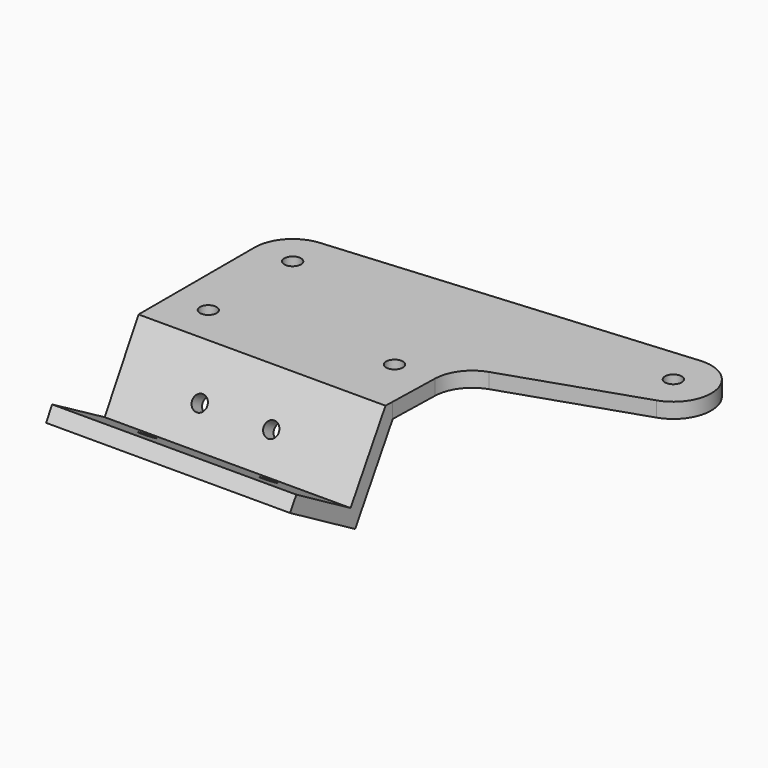
from build123d import *

# Parameters (mm, degrees)
F0_R     = 5.5
F1_DEPTH = 10
F3_DEPTH = 137.8111356168
F4_REACH = 250.1802781517
F5_R     = 5
F6_DEPTH = 152.6664515987
F7_R     = 5
F8_DEPTH = 35.9817621135


with BuildPart() as f1:
    # F0 (on Top) → F1 (new body)
    with BuildSketch(Plane.XY):
        with BuildLine():
            ThreePointArc((-114.9011806829, 81.9265817605), (-131.2129171427, 73.936702076), (-137.8111356168, 57.0141007194))
            Line((-137.8111356168, 57.0141007194), (-137.8111356168, -32.9858992806))
            Line((-137.8111356168, -32.9858992806), (25.1888643832, -32.9858992806))
            Line((25.1888643832, -32.9858992806), (26.0714058339, 0.8295803985))
            ThreePointArc((26.0714058339, 0.8295803985), (30.9682705236, 15.0503307045), (43.1380721252, 23.8880313122))
            Line((43.1380721252, 23.8880313122), (130.3572190405, 53.0392771455))
            ThreePointArc((130.3572190405, 53.0392771455), (146.9184021007, 81.7933335256), (120.3423502221, 101.6624555296))
            Line((120.3423502221, 101.6624555296), (-114.9011806829, 81.9265817605))
        make_face()
        with Locations((-112.8111356168, -12.4858992806)):
            Circle(F0_R, mode=Mode.SUBTRACT)
        Circle(F0_R, mode=Mode.SUBTRACT)
        with Locations((-112.8111356168, 57.0141007194)):
            Circle(F0_R, mode=Mode.SUBTRACT)
        with Locations((122.4323952882, 76.7499744885)):
            Circle(F0_R, mode=Mode.SUBTRACT)
    extrude(amount=F1_DEPTH)

    # F2 (on Right) → F3 (join, through all)
    with BuildSketch(Plane.YZ):
        Polygon((-38.7594019725, 10), (-66.6461533184, -38.3012701892), (-109.9474235076, -13.3012701892), (-114.9474235076, -21.9615242271), (-62.9858992806, -51.9615242271), (-32.9858992806, 0), (-32.9858992806, 10), align=None)
    extrude(amount=-F3_DEPTH)

    f4_end = Plane(origin=(25.6301351085, -16.078159441, 5), x_dir=(0.0260898572, 0.9996596017, 0), z_dir=(0.9996596017, -0.0260898572, 0))
    # F2 (on Right) → F4 (join, up to a plane its end follows)
    with BuildSketch(Plane.YZ):
        Polygon((-38.7594019725, 10), (-66.6461533184, -38.3012701892), (-109.9474235076, -13.3012701892), (-114.9474235076, -21.9615242271), (-62.9858992806, -51.9615242271), (-32.9858992806, 0), (-32.9858992806, 10), align=None)
    f4_long = extrude(amount=F4_REACH, mode=Mode.PRIVATE)
    add(split(f4_long, bisect_by=f4_end, keep=Keep.BOTTOM, mode=Mode.PRIVATE))

    # F5 (on face) → F6 (cut, through all)
    with BuildSketch(Plane(origin=(0, -33.3996784983, 19.2833133718), x_dir=(1, 0, 0), z_dir=(0, -0.8660254038, 0.5))):
        with Locations((-84.6435874701, -42.7307449281)):
            Circle(F5_R)
        with Locations((-37.48293221, -42.7307449281)):
            Circle(F5_R)
    extrude(amount=-F6_DEPTH, mode=Mode.SUBTRACT)

    # F7 (on face) → F8 (cut, through all)
    with BuildSketch(Plane(origin=(0, -33.2464748201, -57.584583561), x_dir=(1, 0, 0), z_dir=(0, 0.5, 0.8660254038))):
        with Locations((-97.8111356168, -55.862698704)):
            Circle(F7_R)
        with Locations((-17.8111356168, -55.862698704)):
            Circle(F7_R)
    extrude(amount=-F8_DEPTH, mode=Mode.SUBTRACT)


solid = f1.part
